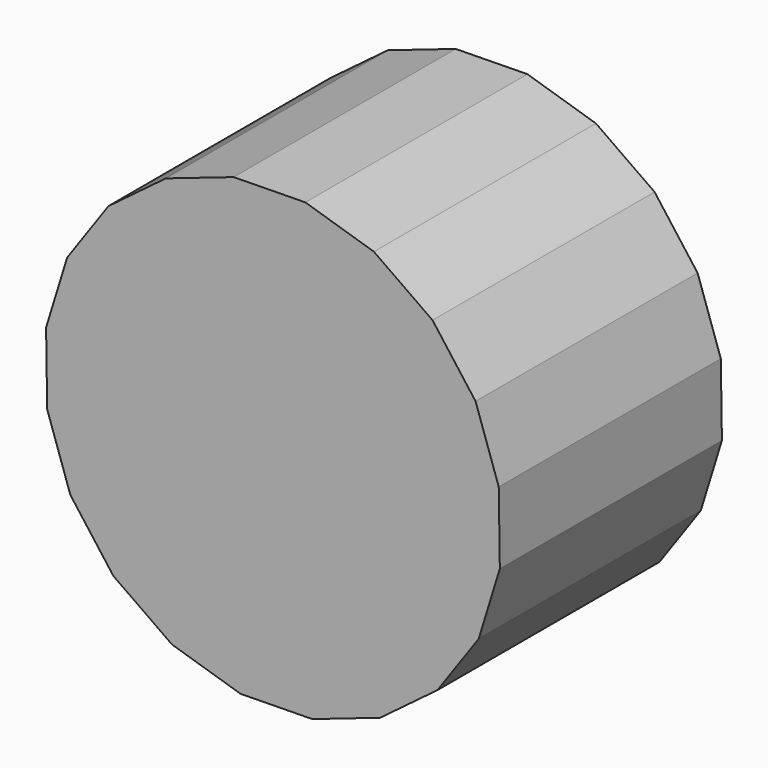
from build123d import *

# Parameters (mm, degrees)
F0_W          = 25.4
F0_H          = 50.8
F1_DEPTH      = 152.4
F2_SIZE       = 12.69999
F4_DEPTH      = 152.401
F6_DEPTH      = 158.75
F6_DEPTH_BACK = 6.35
F7_R          = 129.8689016848
F8_DEPTH      = 2.54
F9_R          = 129.8689016848
F10_DEPTH     = 2.54
F11_R         = 35.7612009526
F12_DEPTH     = 0.0254


# Not quite as in the source:
# - a fillet or chamfer is up to 0.001 mm smaller than in the source, because OpenCascade refuses the exact size


with BuildPart() as f1:
    # F0 (on Front) → F1 (new body)
    with BuildSketch(Plane.XZ):
        Polygon((12.7, -69.7859264541), (25.4, -69.7859264541), (35.1287644276, -61.6225238111), (54.5862932828, -45.2957185251), (64.3150577104, -37.1323158821), (66.5203895668, -24.6252574188), (70.9310532796, 0.3888595077), (73.1363851359, 12.8959179709), (66.7863851359, 23.894440599), (54.0863851359, 45.8914858551), (47.7363851359, 56.8900084832), (35.8022888519, 61.2336643034), (15.5788562807, 68.5943917941), (11.934096284, 69.9209759439), (0, 74.2646317641), (-11.934096284, 69.9209759439), (-35.8022888519, 61.2336643034), (-47.7363851359, 56.8900084832), (-54.0863851359, 45.8914858551), (-66.7863851359, 23.894440599), (-73.1363851359, 12.8959179709), (-70.9310532796, 0.3888595077), (-66.5203895668, -24.6252574188), (-64.3150577104, -37.1323158821), (-54.5862932828, -45.2957185251), (-35.1287644276, -61.6225238111), (-25.4, -69.7859264541), (-12.7, -69.7859264541), align=None)
        Polygon((-110.7804756482, 49.294440599), (-66.7863851359, 23.894440599), (-54.0863851359, 45.8914858551), (-98.0804756482, 71.2914858551), align=None)
        Polygon((-53.1769121329, 108.9700494394), (-35.8022888519, 61.2336643034), (-11.934096284, 69.9209759439), (-29.3087195649, 117.6573610798), align=None)
        Polygon((15.5788562807, 68.5943917941), (35.8022888519, 61.2336643034), (53.1769121329, 108.9700494394), (29.3087195649, 117.6573610798), (13.5150577104, 74.2646317641), align=None)
        Polygon((54.0863851359, 45.8914858551), (66.7863851359, 23.894440599), (110.7804756482, 49.294440599), (98.0804756482, 71.2914858551), align=None)
        Polygon((70.9310532796, 0.3888595077), (66.5203895668, -24.6252574188), (116.5486234198, -33.4465848443), (120.9592871326, -8.4324679178), align=None)
        Polygon((54.5862932828, -45.2957185251), (35.1287644276, -61.6225238111), (67.7823749997, -100.5375815216), (87.2399038549, -84.2107762355), align=None)
        with Locations((0, -95.1859264541)):
            Rectangle(F0_W, F0_H)
        Polygon((-67.7823749997, -100.5375815216), (-35.1287644276, -61.6225238111), (-54.5862932828, -45.2957185251), (-87.2399038549, -84.2107762355), align=None)
        Polygon((-116.5486234198, -33.4465848443), (-66.5203895668, -24.6252574188), (-70.9310532796, 0.3888595077), (-120.9592871326, -8.4324679178), align=None)
    extrude(amount=F1_DEPTH)

    # F2 (size 12.7 in the source; OpenCascade refuses exactly that, so slightly less here)
    f2_edges = [f1.edges().sort_by_distance(p)[0] for p in [
        (54.086385, -76.2, 45.891486),
        (12.7, -76.2, -69.785926),
        (-66.786385, -76.2, 23.894441),
        (54.586293, -76.2, -45.295719),
        (-35.802289, -76.2, 61.233664),
        (-66.52039, -76.2, -24.625257),
        (70.931053, -76.2, 0.38886),
        (-35.128764, -76.2, -61.622524),
    ]]
    chamfer(f2_edges, length=F2_SIZE)

    # F3 (on face) → F4 (cut, through all)
    with BuildSketch(Plane.XZ.offset(152.4)):
        Polygon((-3.6661742094, -6.35), (3.6661742094, -6.35), (7.3323484187, 0), (3.6661742094, 6.35), (-3.6661742094, 6.35), (-7.3323484187, 0), align=None)
    extrude(amount=-F4_DEPTH, mode=Mode.SUBTRACT)


with BuildPart() as f6:
    # F5 (on face) → F6 (new body, two sides)
    with BuildSketch(Plane.XZ.offset(152.4)) as f6_sk:
        Polygon((-122.3742804365, 60.0141262379), (-134.9302417462, 19.261093499), (-134.2782908794, -23.3773492715), (-120.4822453295, -63.7274542157), (-94.8925581576, -97.839471926), (-60.0141262379, -122.3742804365), (-19.261093499, -134.9302417462), (23.3773492715, -134.2782908794), (63.7274542157, -120.4822453295), (97.839471926, -94.8925581576), (122.3742804365, -60.0141262379), (134.9302417462, -19.261093499), (134.2782908794, 23.3773492715), (120.4822453295, 63.7274542157), (94.8925581576, 97.839471926), (60.0141262379, 122.3742804365), (19.261093499, 134.9302417462), (-23.3773492715, 134.2782908794), (-63.7274542157, 120.4822453295), (-97.839471926, 94.8925581576), align=None)
        Polygon((58.9592475765, -115.7140386904), (20.3159721604, -128.27), (-20.3159721604, -128.27), (-58.9592475765, -115.7140386904), (-91.8311810466, -91.8311810466), (-115.7140386904, -58.9592475765), (-128.27, -20.3159721604), (-128.27, 20.3159721604), (-115.7140386904, 58.9592475765), (-91.8311810466, 91.8311810466), (-58.9592475765, 115.7140386904), (-20.3159721604, 128.27), (20.3159721604, 128.27), (58.9592475765, 115.7140386904), (91.8311810466, 91.8311810466), (115.7140386904, 58.9592475765), (128.27, 20.3159721604), (128.27, -20.3159721604), (115.7140386904, -58.9592475765), (91.8311810466, -91.8311810466), align=None, mode=Mode.SUBTRACT)
    extrude(amount=-F6_DEPTH)
    extrude(f6_sk.sketch, amount=F6_DEPTH_BACK)

    # F7 (on face) → F8 (join)
    with BuildSketch(Plane.XZ.offset(158.75)):
        Circle(F7_R)
    extrude(amount=-F8_DEPTH)

    # F9 (on face) → F10 (join)
    with BuildSketch(Plane(origin=(0, 6.35, 0), x_dir=(-1, 0, 0), z_dir=(0, 1, 0))):
        Circle(F9_R)
    extrude(amount=-F10_DEPTH)

    # F11 (on face) → F12 (cut)
    with BuildSketch(Plane(origin=(0, 6.35, 0), x_dir=(-1, 0, 0), z_dir=(0, 1, 0))):
        Circle(F11_R)
    extrude(amount=-F12_DEPTH, mode=Mode.SUBTRACT)


solid = Compound([f1.part, f6.part])
